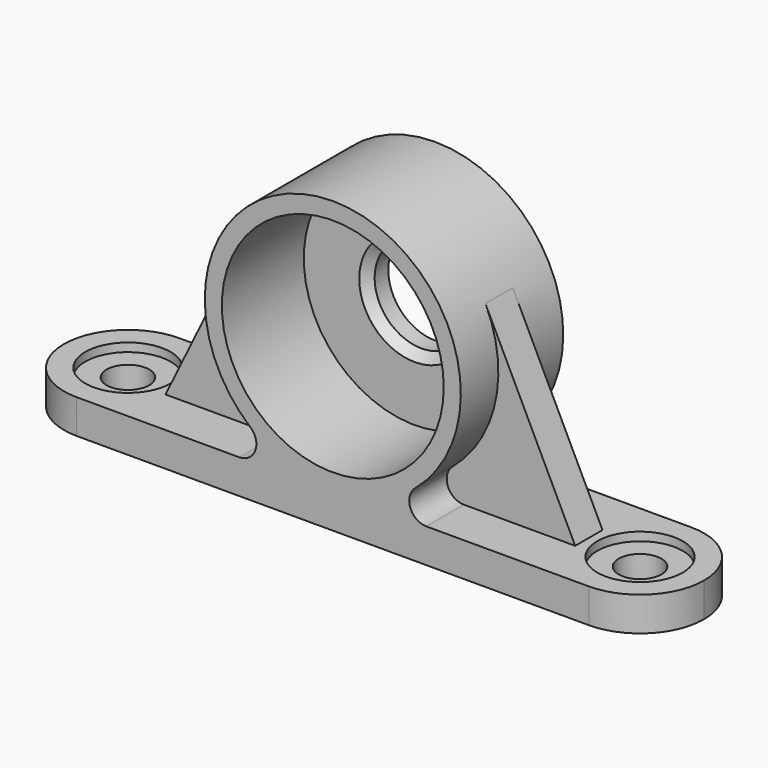
from build123d import *

# Parameters (mm, degrees)
F2_DEPTH       = 7.5
F3_R           = 13
F4_DEPTH       = 12
F5_R           = 5.5
F6_DEPTH       = 15.001
F7_R           = 7.49999
F9_D           = 5
F9_CBORE_D     = 10
F9_CBORE_DEPTH = 1
F11_DEPTH      = 2
F12_SIZE       = 1


# Not quite as in the source:
# - a fillet or chamfer is up to 0.001 mm smaller than in the source, because OpenCascade refuses the exact size


with BuildPart() as f2:
    # F1 (on Front) → F2 (new body, symmetric)
    with BuildSketch(Plane.XZ):
        with BuildLine():
            Line((-37.5, 0), (0, 0))
            Line((0, 0), (37.5, 0))
            Line((37.5, 0), (37.5, 4))
            Line((37.5, 4), (10.9544511501, 4))
            ThreePointArc((10.9544511501, 4), (9.0757782768, 5.3140056594), (9.6656921913, 7.5294117647))
            ThreePointArc((9.6656921913, 7.5294117647), (14.0900465494, 24.1449575543), (0, 34))
            ThreePointArc((0, 34), (-14.0900465494, 24.1449575543), (-9.6656921913, 7.5294117647))
            ThreePointArc((-9.6656921913, 7.5294117647), (-9.0757782768, 5.3140056594), (-10.9544511501, 4))
            Line((-10.9544511501, 4), (-37.5, 4))
            Line((-37.5, 4), (-37.5, 0))
        make_face()
    extrude(amount=F2_DEPTH, both=True)

    # F3 (on face) → F4 (cut)
    with BuildSketch(Plane.XZ.offset(7.5)):
        with Locations((0, 19)):
            Circle(F3_R)
    extrude(amount=-F4_DEPTH, mode=Mode.SUBTRACT)

    # F5 (on face) → F6 (cut, through all)
    with BuildSketch(Plane(origin=(0, 7.5, 0), x_dir=(-1, 0, 0), z_dir=(0, 1, 0))):
        with Locations((0, 19)):
            Circle(F5_R)
    extrude(amount=-F6_DEPTH, mode=Mode.SUBTRACT)

    # F7 (radius 7.5 in the source; OpenCascade refuses exactly that, so slightly less here)
    f7_edges = [f2.edges().sort_by_distance(p)[0] for p in [
        (37.5, -7.5, 2),
        (37.5, 7.5, 2),
        (-37.5, -7.5, 2),
        (-37.5, 7.5, 2),
    ]]
    fillet(f7_edges, radius=F7_R)

    # F9 (through all)
    with Locations(Plane.XY.offset(4)):
        with Locations((30, 0), (-30, 0)):
            CounterBoreHole(F9_D / 2, F9_CBORE_D / 2, F9_CBORE_DEPTH)

    # F10 (on Front) → F11 (join, symmetric)
    with BuildSketch(Plane.XZ):
        with BuildLine():
            Line((10.9544511501, 4), (24, 4))
            Line((24, 4), (13.4831460674, 25.5730337079))
            ThreePointArc((13.4831460674, 25.5730337079), (14.6751576274, 15.8952055444), (9.6656921913, 7.5294117647))
            ThreePointArc((9.6656921913, 7.5294117647), (9.0757782768, 5.3140056594), (10.9544511501, 4))
        make_face()
    extrude(amount=F11_DEPTH, both=True)

    # F12
    f12_edges = [f2.edges().sort_by_distance(p)[0] for p in [
        (5.5, 4.5, 19),
    ]]
    chamfer(f12_edges, length=F12_SIZE)

    # F13: F2 across plane


with BuildPart() as f2_1:
    add(f2.part)
    add(f2.part.mirror(Plane.YZ))


solid = f2_1.part
